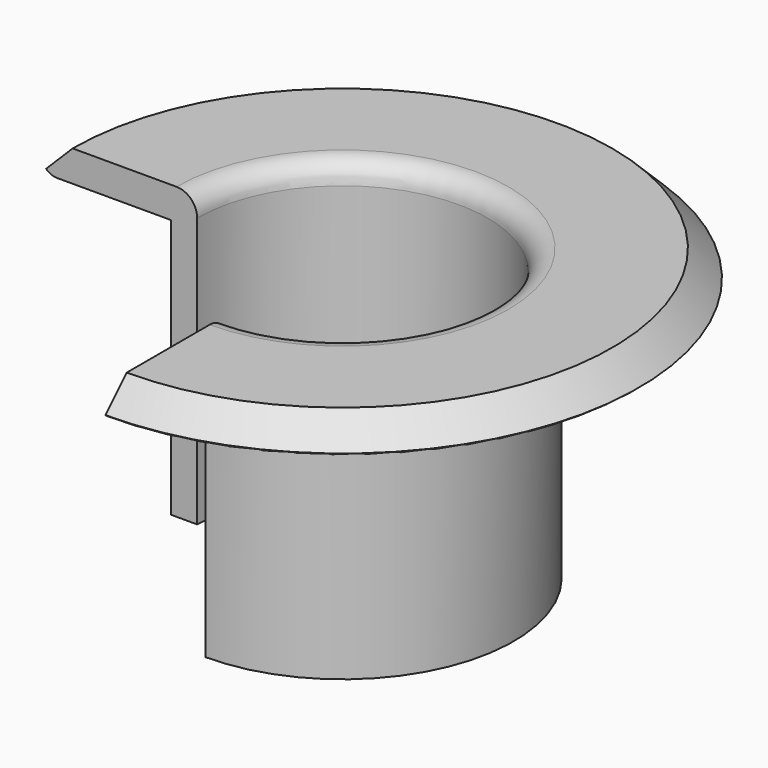
from build123d import *

# Parameters (mm, degrees)
F1_ANGLE    = 270
F2_R        = 1.5
F3_T2_ANGLE = 300.5959645066
F4_R        = 2


# Not quite as in the source:
# - a fillet or chamfer that OpenCascade refuses, or shapes differently, is made with other operations: its cross-section is extruded or revolved along the edge and cut away or added


with BuildPart() as f1:
    # F0 (on Front) → F1 (revolve)
    with BuildSketch(Plane.XZ):
        Polygon((-2.5, 0), (0, 0), (0, 28), (-15, 28), (-15, 25), (-12.5, 25), (-2.5, 25), align=None)
    revolve(axis=Axis((14, 0, -3.1492561102), (0, 0, -1)), revolution_arc=F1_ANGLE)

    # F2
    f2_edges = [f1.edges().sort_by_distance(p)[0] for p in [
        (34.506097, 20.506097, 25),
    ]]
    fillet(f2_edges, radius=F2_R)

    # F3: chamfer of 3 on 1 edges, made by hand

    # F3_s1 → F3_t2 (revolve, cut)
    with BuildSketch(Plane(origin=(0.974554854, -3.562865531, 0), x_dir=(0, 0, 1), z_dir=(0.2638390816, -0.9645667105, 0))):
        Polygon((25, 15.496066053), (28, 12.496066053), (28, 15.496066053), align=None)
    revolve(axis=Axis((14, 0, 28), (0, 0, -1)), revolution_arc=F3_T2_ANGLE, mode=Mode.SUBTRACT)

    # F4
    f4_edges = [f1.edges().sort_by_distance(p)[0] for p in [
        (23.899495, 9.899495, 28),
    ]]
    fillet(f4_edges, radius=F4_R)


solid = f1.part
